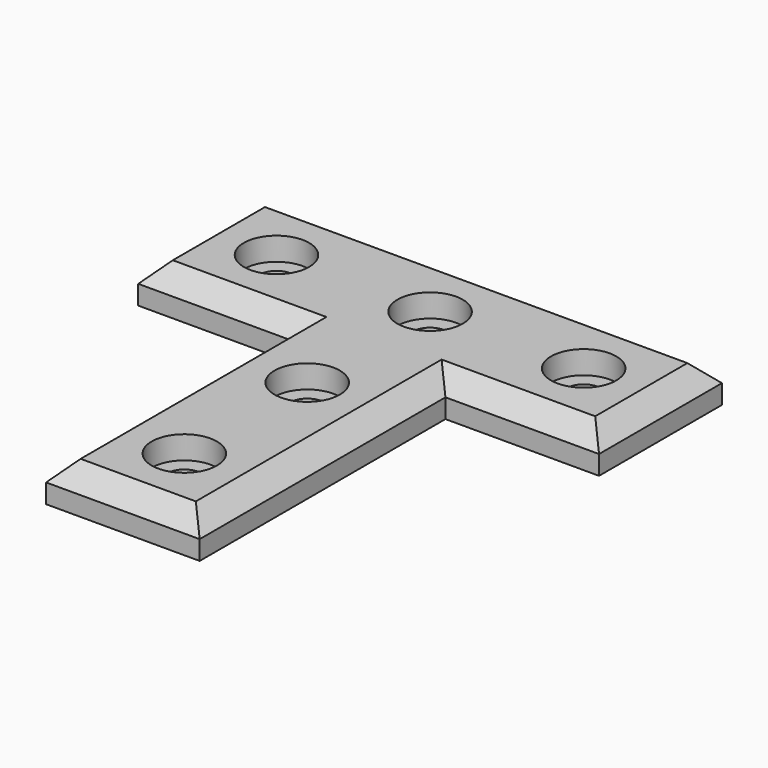
from build123d import *

# Parameters (mm, degrees)
F0_R     = 2.25
F1_DEPTH = 5
F2_SIZE  = 2.5
F3_R     = 4.25
F3_R_2   = 2.25
F4_DEPTH = 3


with BuildPart() as f1:
    # F0 (on Top) → F1 (new body)
    with BuildSketch(Plane.XY):
        Polygon((-10, -50), (0, -50), (10, -50), (10, -10), (30, -10), (30, 10), (0, 10), (-30, 10), (-30, -10), (-10, -10), align=None)
        with Locations((0, -40)):
            Circle(F0_R, mode=Mode.SUBTRACT)
        with Locations((-20, 0)):
            Circle(F0_R, mode=Mode.SUBTRACT)
        with Locations((0, -20)):
            Circle(F0_R, mode=Mode.SUBTRACT)
        Circle(F0_R, mode=Mode.SUBTRACT)
        with Locations((20, 0)):
            Circle(F0_R, mode=Mode.SUBTRACT)
    extrude(amount=F1_DEPTH)

    # F2
    f2_edges = [f1.edges().sort_by_distance(p)[0] for p in [
        (0, -50, 5),
        (10, -30, 5),
        (20, -10, 5),
        (30, 0, 5),
        (0, 10, 5),
        (-30, 0, 5),
        (-20, -10, 5),
        (-10, -30, 5),
    ]]
    chamfer(f2_edges, length=F2_SIZE)

    # F3 (on face) → F4 (cut)
    with BuildSketch(Plane.XY.offset(5)):
        with Locations((-20, 0)):
            Circle(F3_R)
        with Locations((-20, 0)):
            Circle(F3_R_2, mode=Mode.SUBTRACT)
        Circle(F3_R)
        Circle(F3_R_2, mode=Mode.SUBTRACT)
        with Locations((20, 0)):
            Circle(F3_R)
        with Locations((20, 0)):
            Circle(F3_R_2, mode=Mode.SUBTRACT)
        with Locations((0, -20)):
            Circle(F3_R)
        with Locations((0, -20)):
            Circle(F3_R_2, mode=Mode.SUBTRACT)
        with Locations((0, -40)):
            Circle(F3_R)
        with Locations((0, -40)):
            Circle(F3_R_2, mode=Mode.SUBTRACT)
    extrude(amount=-F4_DEPTH, mode=Mode.SUBTRACT)


solid = f1.part
